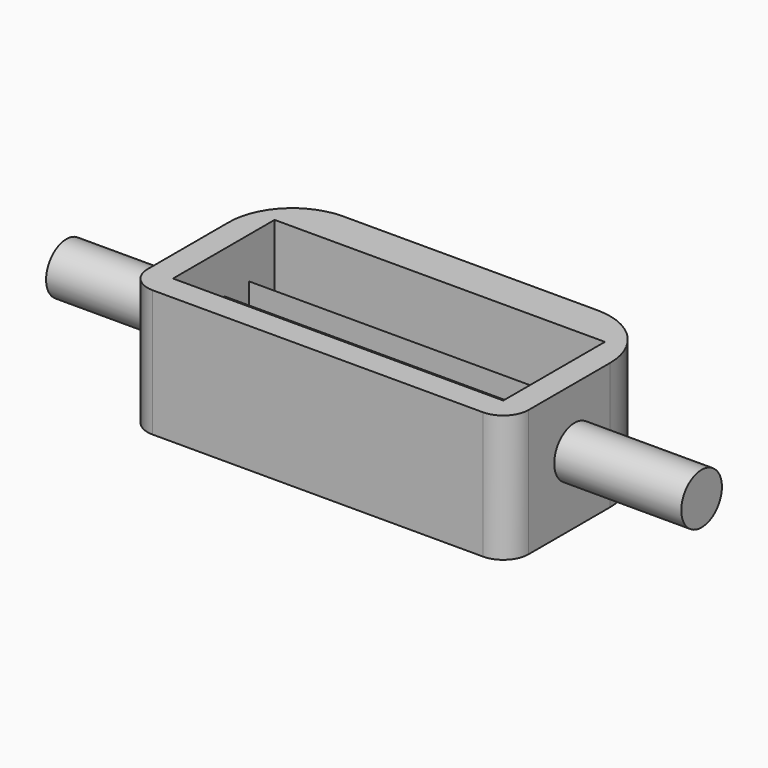
from build123d import *

# Parameters (mm, degrees)
F0_W         = 76.2
F0_H         = 38.1
F1_DEPTH     = 25.4
F2_R         = 12.7
F3_R         = 5.08
F4_R         = 5.08
F5_DEPTH     = 25.4
F6_R         = 5.08
F7_DEPTH     = 25.4
F8_W         = 66.04
F8_H         = 25.4
F9_DEPTH     = 19.05
F10_W        = 66.04
F10_H        = 3.175
F11_DEPTH    = 12.7
F12_T1_DEPTH = 66.04
F12_T6_DEPTH = 66.04


# Not quite as in the source:
# - a fillet or chamfer that OpenCascade refuses, or shapes differently, is made with other operations: its cross-section is extruded or revolved along the edge and cut away or added


with BuildPart() as f1:
    # F0 (on Top) → F1 (new body)
    with BuildSketch(Plane.XY):
        with Locations((-1.7044725776, 2.5065781057)):
            Rectangle(F0_W, F0_H)
    extrude(amount=F1_DEPTH)

    # F2
    f2_edges = [f1.edges().sort_by_distance(p)[0] for p in [
        (-39.804473, 21.556578, 12.7),
        (36.395527, 21.556578, 12.7),
    ]]
    fillet(f2_edges, radius=F2_R)

    # F3
    f3_edges = [f1.edges().sort_by_distance(p)[0] for p in [
        (-39.804473, -16.543422, 12.7),
        (36.395527, -16.543422, 12.7),
    ]]
    fillet(f3_edges, radius=F3_R)

    # F4 (on face) → F5 (join)
    with BuildSketch(Plane(origin=(-39.8044725776, 0, 0), x_dir=(0, -1, 0), z_dir=(-1, 0, 0))):
        with Locations((0, 12.7)):
            Circle(F4_R)
    extrude(amount=F5_DEPTH)

    # F6 (on face) → F7 (join)
    with BuildSketch(Plane.YZ.offset(36.3955274224)):
        with Locations((0, 13.3897410706)):
            Circle(F6_R)
    extrude(amount=F7_DEPTH)

    # F8 (on face) → F9 (cut)
    with BuildSketch(Plane.XY.offset(25.4)):
        with Locations((-1.7044725776, 1.2365781057)):
            Rectangle(F8_W, F8_H)
    extrude(amount=-F9_DEPTH, mode=Mode.SUBTRACT)

    # F10 (on face) → F11 (join)
    with BuildSketch(Plane.XY.offset(6.35)):
        with Locations((-1.7044725776, 9.1740781057)):
            Rectangle(F10_W, F10_H)
        with Locations((-1.7044725776, 2.8240781057)):
            Rectangle(F10_W, F10_H)
        with Locations((-1.7044725776, -3.5259218943)):
            Rectangle(F10_W, F10_H)
        with Locations((-1.7044725776, -9.8759218943)):
            Rectangle(F10_W, F10_H)
    extrude(amount=F11_DEPTH)

    # F12: chamfer of 5.08 on 4 edges, made by hand

    # F12_s2 → F12_t1 (cut)
    with BuildSketch(Plane.YZ.offset(-34.7244725776)):
        Polygon((5.6815781057, 19.05), (10.7615781057, 13.97), (10.7615781057, 19.05), align=None)
        Polygon((-0.6684218943, 19.05), (4.4115781057, 13.97), (4.4115781057, 19.05), align=None)
        Polygon((-7.0184218943, 19.05), (-1.9384218943, 13.97), (-1.9384218943, 19.05), align=None)
    extrude(amount=F12_T1_DEPTH, mode=Mode.SUBTRACT)


with BuildPart() as f12_tool4:
    # F12_s5 → F12_t6 (new body)
    with BuildSketch(Plane.YZ.offset(31.3155274224)):
        Polygon((-13.3684218943, 19.05), (-8.2884218943, 13.97), (-8.2884218943, 19.05), align=None)
    extrude(amount=-F12_T6_DEPTH)

    split(bisect_by=Plane.XZ.offset(11.4634218943), keep=Keep.BOTTOM)


with BuildPart() as f1_1:
    add(f1.part)

    # F12_t3: cut F12_tool4
    add(f12_tool4.part, mode=Mode.SUBTRACT)


solid = f1_1.part
